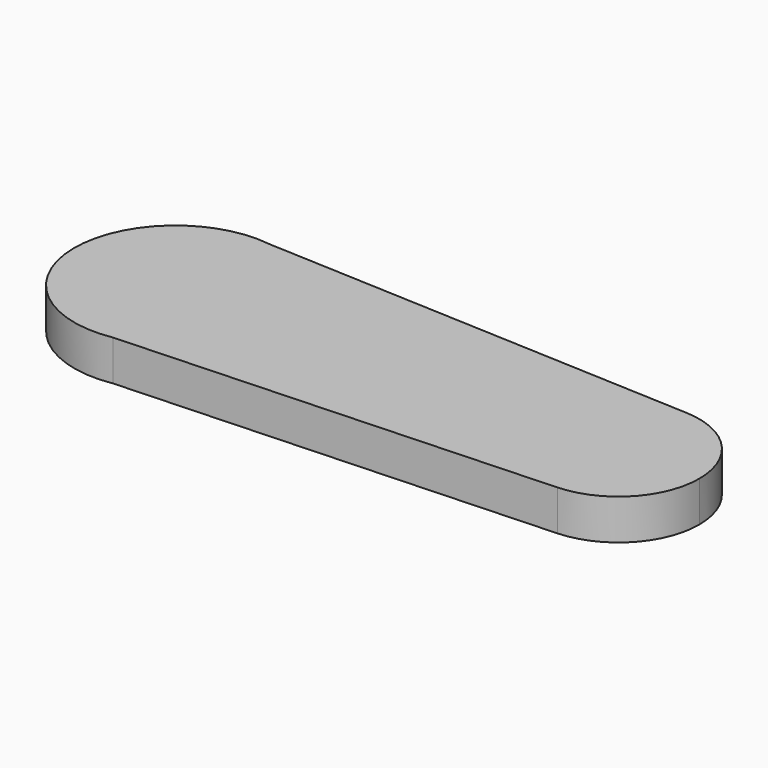
from build123d import *

# Parameters (mm, degrees)
F1_DEPTH = 10


# Not quite as in the source:
# - the program builds the solid bodies; features that only make, move or delete a surface that nothing else refers to are left out


with BuildPart() as f1:
    # F0 (on Top) → F1 (new body)
    with BuildSketch(Plane.XY):
        with BuildLine():
            ThreePointArc((4.2686762947, -24.6328724003), (19.1274267397, -16.0978739688), (25, 0))
            ThreePointArc((25, 0), (18.8537485405, 16.4175566383), (3.4371067222, 24.7625987606))
            ThreePointArc((3.4371067222, 24.7625987606), (-24.9964580647, -0.42081376), (4.2686762947, -24.6328724003))
        make_face()
        with BuildLine():
            ThreePointArc((110.4968080295, 19.9800743296), (95.7812936366, 14.4542523825), (89.6042668357, 0))
            ThreePointArc((89.6042668357, 0), (95.7750082208, -14.4482388602), (110.4794274519, -19.9808431728))
            ThreePointArc((110.4794274519, -19.9808431728), (124.0525056959, -13.8292586149), (129.6042668357, 0))
            ThreePointArc((129.6042668357, 0), (124.0585192182, 13.8229731991), (110.4968080295, 19.9800743296))
        make_face()
        with BuildLine():
            Line((89.6042668357, 0), (25, 0))
            ThreePointArc((25, 0), (19.1274267397, -16.0978739688), (4.2686762947, -24.6328724003))
            Line((4.2686762947, -24.6328724003), (110.4794274519, -19.9808431728))
            ThreePointArc((110.4794274519, -19.9808431728), (95.7750082208, -14.4482388602), (89.6042668357, 0))
        make_face()
        with BuildLine():
            ThreePointArc((3.4371067222, 24.7625987606), (18.8537485405, 16.4175566383), (25, 0))
            Line((25, 0), (89.6042668357, 0))
            ThreePointArc((89.6042668357, 0), (95.7812936366, 14.4542523825), (110.4968080295, 19.9800743296))
            Line((110.4968080295, 19.9800743296), (3.4371067222, 24.7625987606))
        make_face()
    extrude(amount=F1_DEPTH)


solid = f1.part
